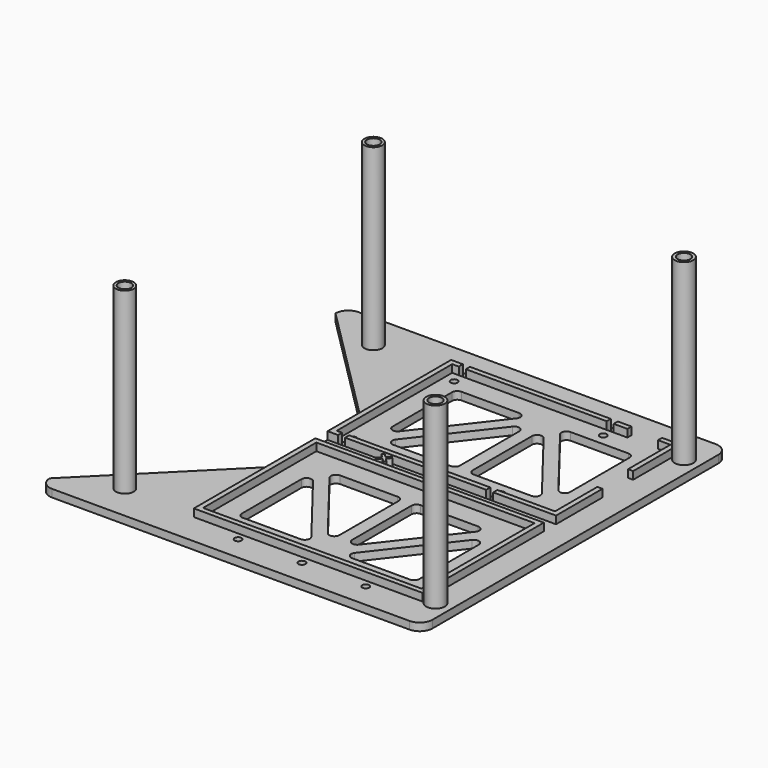
from build123d import *

# Parameters (mm, degrees)
F0_W         = 150
F0_H         = 150
F1_DEPTH     = 3
F2_W         = 89.5
F2_H         = 60.5
F2_W_2       = 85.5
F2_H_2       = 56.5
F3_DEPTH     = 3
F4_W         = 12
F4_H         = 2
F4_W_2       = 2
F4_H_2       = 15
F5_DEPTH     = 3
F6_R         = 5
F7_W         = 89.5
F7_H         = 59.5
F7_W_2       = 85.5
F7_H_2       = 55.5
F8_DEPTH     = 3
F9_R         = 3.6271227465
F9_R_2       = 2.5
F9_R_3       = 3.5
F10_DEPTH    = 70
F12_DEPTH    = 3
F13_R        = 2.5
F13_R_2      = 28.6222607242
F13_R_3      = 34.4815327899
F13_R_4      = 36.1444775831
F14_DEPTH    = 25
F16_DEPTH    = 25
F17_T1_DEPTH = 3
F18_R        = 1.375
F19_DEPTH    = 25
F20_W        = 2.75
F20_H        = 2
F21_DEPTH    = 25
F23_R        = 1.375
F24_DEPTH    = 25
F26_DEPTH    = 25


# Not quite as in the source:
# - a fillet or chamfer that OpenCascade refuses, or shapes differently, is made with other operations: its cross-section is extruded or revolved along the edge and cut away or added


with BuildPart() as f1:
    # F0 (on Top) → F1 (new body)
    with BuildSketch(Plane.XY):
        Rectangle(F0_W, F0_H)
    extrude(amount=F1_DEPTH)

    # F2 (on face) → F3 (join)
    with BuildSketch(Plane.XY.offset(3)):
        with Locations((20.25, 33.25)):
            Rectangle(F2_W, F2_H)
        with Locations((20.25, 33.25)):
            Rectangle(F2_W_2, F2_H_2, mode=Mode.SUBTRACT)
    extrude(amount=F3_DEPTH)

    # F4 (on face) → F5 (cut)
    with BuildSketch(Plane.XY.offset(6)):
        with Locations((52.15, 62.5)):
            Rectangle(F4_W, F4_H)
        with Locations((64, 33.25)):
            Rectangle(F4_W_2, F4_H_2)
    extrude(amount=-F5_DEPTH, mode=Mode.SUBTRACT)

    # F6
    f6_edges = [f1.edges().sort_by_distance(p)[0] for p in [
        (-75, 75, 1.5),
        (75, 75, 1.5),
        (75, -75, 1.5),
        (-75, -75, 1.5),
    ]]
    fillet(f6_edges, radius=F6_R)

    # F7 (on face) → F8 (join)
    with BuildSketch(Plane.XY.offset(3)):
        with Locations((20.25, -32.75)):
            Rectangle(F7_W, F7_H)
        with Locations((20.25, -32.75)):
            Rectangle(F7_W_2, F7_H_2, mode=Mode.SUBTRACT)
    extrude(amount=F8_DEPTH)

    # F9 (on face) → F10 (join)
    with BuildSketch(Plane.XY.offset(3)):
        with Locations((68.8578643763, 60.8578643763)):
            Circle(F9_R)
        with Locations((68.8578643763, 60.8578643763)):
            Circle(F9_R_2, mode=Mode.SUBTRACT)
        with Locations((68.8578643763, -60.8578643763)):
            Circle(F9_R)
        with Locations((68.8578643763, -60.8578643763)):
            Circle(F9_R_2, mode=Mode.SUBTRACT)
        with Locations((-52.8578643763, 60.8578643763)):
            Circle(F9_R_3)
        with Locations((-52.8578643763, 60.8578643763)):
            Circle(F9_R_2, mode=Mode.SUBTRACT)
        with Locations((-52.8578643763, -60.8578643763)):
            Circle(F9_R_3)
        with Locations((-52.8578643763, -60.8578643763)):
            Circle(F9_R_2, mode=Mode.SUBTRACT)
    extrude(amount=F10_DEPTH)

    # F11 (on face) → F12 (join)
    with BuildSketch(Plane.XY.offset(3)):
        Polygon((-1.4142135624, 2.1213203436), (-2.1213203436, 1.4142135624), (-0.7071067812, 0), (-2.1213203436, -1.4142135624), (-1.4142135624, -2.1213203436), (0, -0.7071067812), (1.4142135624, -2.1213203436), (2.1213203436, -1.4142135624), (0.7071067812, 0), (2.1213203436, 1.4142135624), (1.4142135624, 2.1213203436), (0, 0.7071067812), align=None)
    extrude(amount=F12_DEPTH)

    # F13 (on face) → F14 (cut)
    with BuildSketch(Plane.XY.offset(3)):
        with Locations((-52.8578643763, 60.8578643763)):
            Circle(F13_R)
        with Locations((662.2217056946, 102.264947845)):
            Circle(F13_R_2)
        with Locations((693.5295645663, -597.344861617)):
            Circle(F13_R_3)
        with Locations((-44.6129470708, -626.2444101651)):
            Circle(F13_R_4)
        with Locations((68.8578643763, 60.8578643763)):
            Circle(F13_R)
        with Locations((68.8578643763, -60.8578643763)):
            Circle(F13_R)
        with Locations((-52.8578643763, -60.8578643763)):
            Circle(F13_R)
    extrude(amount=-F14_DEPTH, mode=Mode.SUBTRACT)

    # F15 (on face) → F16 (cut)
    with BuildSketch(Plane.XY.offset(3)):
        Polygon((-24.5, 19.5), (-75, 70), (-75, -70), (-24.5, -19.5), align=None)
    extrude(amount=-F16_DEPTH, mode=Mode.SUBTRACT)

    # F17: fillet of radius 5 on 4 edges, made by hand

    # F17_s2 → F17_t1 (join)
    with BuildSketch(Plane.XY):
        with BuildLine():
            ThreePointArc((-24.5, 17.4289321881), (-24.8806023374, 19.34234935), (-25.9644660941, 20.9644660941))
            Line((-25.9644660941, 20.9644660941), (-24.5, 19.5))
            Line((-24.5, 19.5), (-24.5, 17.4289321881))
        make_face()
        with BuildLine():
            ThreePointArc((-25.9644660941, -20.9644660941), (-24.8806023374, -19.34234935), (-24.5, -17.4289321881))
            Line((-24.5, -17.4289321881), (-24.5, -19.5))
            Line((-24.5, -19.5), (-25.9644660941, -20.9644660941))
        make_face()
    extrude(amount=F17_T1_DEPTH)

    # F18 (on face) → F19 (cut)
    with BuildSketch(Plane.XY.offset(6)):
        with Locations((-18.5, 57.5)):
            Circle(F18_R)
        with Locations((39.5, 58)):
            Circle(F18_R)
        with Locations((-19, 8.5)):
            Circle(F18_R)
        with Locations((39, 8.5)):
            Circle(F18_R)
    extrude(amount=-F19_DEPTH, mode=Mode.SUBTRACT)

    # F20 (on face) → F21 (cut)
    with BuildSketch(Plane.XY.offset(6)):
        with Locations((-18.525, 62.5)):
            Rectangle(F20_W, F20_H)
        with Locations((39.425, 62.5)):
            Rectangle(F20_W, F20_H)
        with Locations((39.025, 4)):
            Rectangle(F20_W, F20_H)
        with Locations((-19.025, 4)):
            Rectangle(F20_W, F20_H)
    extrude(amount=-F21_DEPTH, mode=Mode.SUBTRACT)

    # F23 (on face) → F24 (cut)
    with BuildSketch(Plane.XY.offset(3)):
        with Locations((-4.75, 0)):
            Circle(F23_R)
        with Locations((20.25, 0)):
            Circle(F23_R)
        with Locations((45.25, 0)):
            Circle(F23_R)
        with Locations((45.25, -65.5)):
            Circle(F23_R)
        with Locations((20.25, -65.5)):
            Circle(F23_R)
        with Locations((-4.75, -65.5)):
            Circle(F23_R)
    extrude(amount=-F24_DEPTH, mode=Mode.SUBTRACT)

    # F25 (on face) → F26 (cut)
    with BuildSketch(Plane.XY.offset(6)):
        with BuildLine():
            Line((48.8800137441, 16.2271423447), (26.3292788436, 45.2489576949))
            ThreePointArc((26.3292788436, 45.2489576949), (24.1013697846, 45.9137135619), (22.75, 44.0218153502))
            Line((22.75, 44.0218153502), (22.75, 15))
            ThreePointArc((22.75, 15), (23.3357864376, 13.5857864376), (24.75, 13))
            Line((24.75, 13), (47.3007349005, 13))
            ThreePointArc((47.3007349005, 13), (49.0971597792, 14.120876769), (48.8800137441, 16.2271423447))
        make_face()
        with BuildLine():
            Line((28.7575768219, 50.2728576553), (51.4207211564, 21.1063762509))
            ThreePointArc((51.4207211564, 21.1063762509), (53.6486302154, 20.4416203838), (55, 22.3335185956))
            Line((55, 22.3335185956), (55, 51.5))
            ThreePointArc((55, 51.5), (54.4142135624, 52.9142135624), (53, 53.5))
            Line((53, 53.5), (30.3368556655, 53.5))
            ThreePointArc((30.3368556655, 53.5), (28.5404307868, 52.379123231), (28.7575768219, 50.2728576553))
        make_face()
        with BuildLine():
            ThreePointArc((-12.5, 53.5), (-13.9142135624, 52.9142135624), (-14.5, 51.5))
            Line((-14.5, 51.5), (-14.5, 22.3335185956))
            ThreePointArc((-14.5, 22.3335185956), (-13.1486302154, 20.4416203838), (-10.9207211564, 21.1063762509))
            Line((-10.9207211564, 21.1063762509), (11.7424231781, 50.2728576553))
            ThreePointArc((11.7424231781, 50.2728576553), (11.9595692132, 52.379123231), (10.1631443345, 53.5))
            Line((10.1631443345, 53.5), (-12.5, 53.5))
        make_face()
        with BuildLine():
            Line((17.75, 15), (17.75, 44.0218153502))
            ThreePointArc((17.75, 44.0218153502), (16.3986302154, 45.9137135619), (14.1707211564, 45.2489576949))
            Line((14.1707211564, 45.2489576949), (-8.3800137441, 16.2271423447))
            ThreePointArc((-8.3800137441, 16.2271423447), (-8.5971597792, 14.120876769), (-6.8007349005, 13))
            Line((-6.8007349005, 13), (15.75, 13))
            ThreePointArc((15.75, 13), (17.1642135624, 13.5857864376), (17.75, 15))
        make_face()
        with BuildLine():
            Line((-14.5, -22.3335185956), (-14.5, -51.5))
            ThreePointArc((-14.5, -51.5), (-13.9142135624, -52.9142135624), (-12.5, -53.5))
            Line((-12.5, -53.5), (10.1631443345, -53.5))
            ThreePointArc((10.1631443345, -53.5), (11.9595692132, -52.379123231), (11.7424231781, -50.2728576553))
            Line((11.7424231781, -50.2728576553), (-10.9207211564, -21.1063762509))
            ThreePointArc((-10.9207211564, -21.1063762509), (-13.1486302154, -20.4416203838), (-14.5, -22.3335185956))
        make_face()
        with BuildLine():
            ThreePointArc((24.75, -13), (23.3357864376, -13.5857864376), (22.75, -15))
            Line((22.75, -15), (22.75, -44.0218153502))
            ThreePointArc((22.75, -44.0218153502), (24.1013697846, -45.9137135619), (26.3292788436, -45.2489576949))
            Line((26.3292788436, -45.2489576949), (48.8800137441, -16.2271423447))
            ThreePointArc((48.8800137441, -16.2271423447), (49.0971597792, -14.120876769), (47.3007349005, -13))
            Line((47.3007349005, -13), (24.75, -13))
        make_face()
        with BuildLine():
            ThreePointArc((53, -53.5), (54.4142135624, -52.9142135624), (55, -51.5))
            Line((55, -51.5), (55, -22.3335185956))
            ThreePointArc((55, -22.3335185956), (53.6486302154, -20.4416203838), (51.4207211564, -21.1063762509))
            Line((51.4207211564, -21.1063762509), (28.7575768219, -50.2728576553))
            ThreePointArc((28.7575768219, -50.2728576553), (28.5404307868, -52.379123231), (30.3368556655, -53.5))
            Line((30.3368556655, -53.5), (53, -53.5))
        make_face()
        with BuildLine():
            Line((17.75, -44.0218153502), (17.75, -15))
            ThreePointArc((17.75, -15), (17.1642135624, -13.5857864376), (15.75, -13))
            Line((15.75, -13), (-6.8007349005, -13))
            ThreePointArc((-6.8007349005, -13), (-8.5971597792, -14.120876769), (-8.3800137441, -16.2271423447))
            Line((-8.3800137441, -16.2271423447), (14.1707211564, -45.2489576949))
            ThreePointArc((14.1707211564, -45.2489576949), (16.3986302154, -45.9137135619), (17.75, -44.0218153502))
        make_face()
    extrude(amount=-F26_DEPTH, mode=Mode.SUBTRACT)


solid = f1.part
